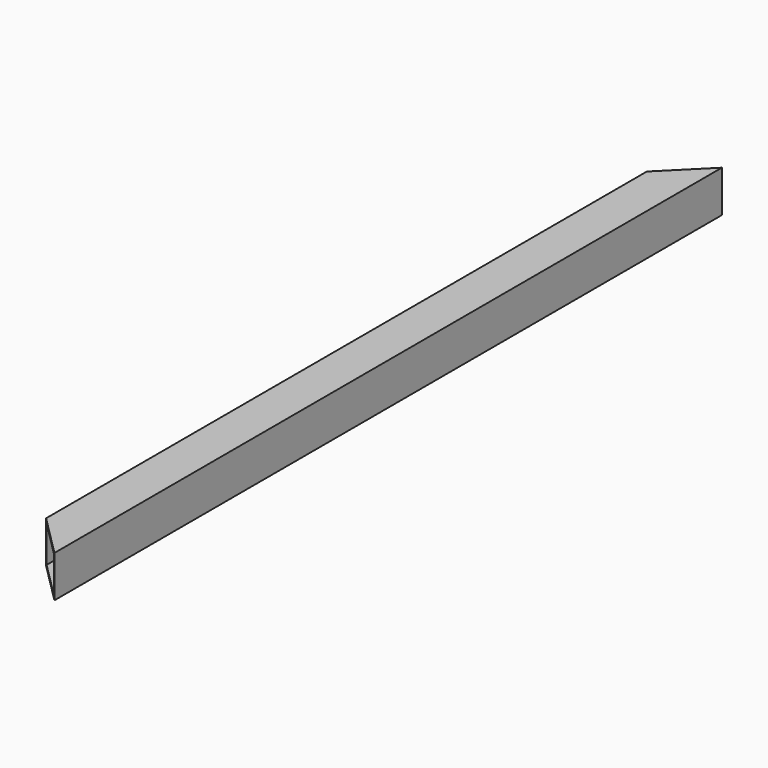
from build123d import *

# Parameters (mm, degrees)
F0_W        = 50
F0_H        = 50
F0_W_2      = 44
F0_H_2      = 44
F1_DEPTH    = 1000
F2_T1_DEPTH = 307.1682987966


# Not quite as in the source:
# - a fillet or chamfer that OpenCascade refuses, or shapes differently, is made with other operations: its cross-section is extruded or revolved along the edge and cut away or added


with BuildPart() as f1:
    # F0 (on Front) → F1 (new body)
    with BuildSketch(Plane.XZ):
        Rectangle(F0_W, F0_H)
        Rectangle(F0_W_2, F0_H_2, mode=Mode.SUBTRACT)
    extrude(amount=F1_DEPTH)

    # F2: chamfer of 50 on 2 edges, made by hand

    # F2_s2 → F2_t1 (cut)
    with BuildSketch(Plane.XY.offset(-153.5841493983)):
        Polygon((-25, -950), (25, -1000), (-25, -1000), align=None)
        Polygon((-25, -50), (25, 0), (-25, 0), align=None)
    extrude(amount=F2_T1_DEPTH, mode=Mode.SUBTRACT)


solid = f1.part
